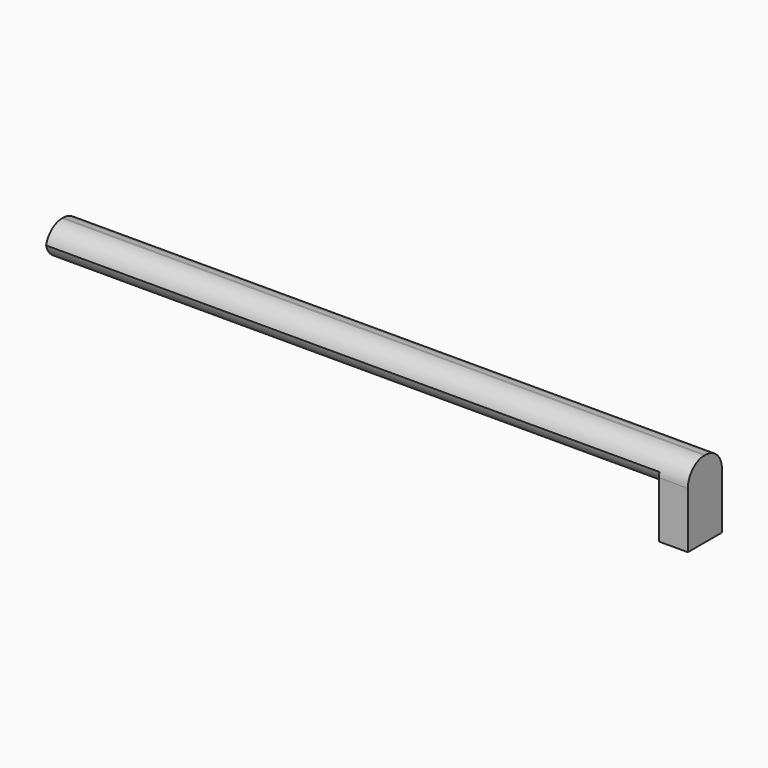
from build123d import *

# Parameters (mm, degrees)
F0_W     = 3.3884318545
F0_H     = 5.3184241988
F1_DEPTH = 5
F2_F1_R  = 2.4142135624
F2_F2_R  = 2.4142135624
F2_F3_R  = 2.4142135624
F2_F4_R  = 2.4142135624
F3_SCALE = 0.125


with BuildPart() as f1:
    # F0 (on Front) → F1 (new body)
    with BuildSketch(Plane.XZ):
        Polygon((17.4084361643, 12.4068003497), (-58.0119900405, 12.4068003497), (-58.0119900405, 8.7094834889), (14.0200043097, 8.7094834889), (17.4084361643, 8.7094834889), align=None)
        with Locations((15.714220237, 6.0502713895)):
            Rectangle(F0_W, F0_H)
    extrude(amount=F1_DEPTH)

    # F2: fillet of radius 2.4142135624 on 4 edges, made by hand

    # F2_f1
    f2_f1_edges = [f1.edges().sort_by_distance(p)[0] for p in [
        (-21.9959928654, 0, 8.7094834889),
    ]]
    fillet(f2_f1_edges, radius=F2_F1_R)

    # F2_f2
    f2_f2_edges = [f1.edges().sort_by_distance(p)[0] for p in [
        (-21.9959928654, -5, 8.7094834889),
    ]]
    fillet(f2_f2_edges, radius=F2_F2_R)

    # F2_f3
    f2_f3_edges = [f1.edges().sort_by_distance(p)[0] for p in [
        (-20.3017769381, 0, 12.4068003497),
    ]]
    fillet(f2_f3_edges, radius=F2_F3_R)

    # F2_f4
    f2_f4_edges = [f1.edges().sort_by_distance(p)[0] for p in [
        (-20.3017769381, -5, 12.4068003497),
    ]]
    fillet(f2_f4_edges, radius=F2_F4_R)


with BuildPart() as f1_1:
    # F3: moved
    add(f1.part.scale(F3_SCALE))


solid = f1_1.part
